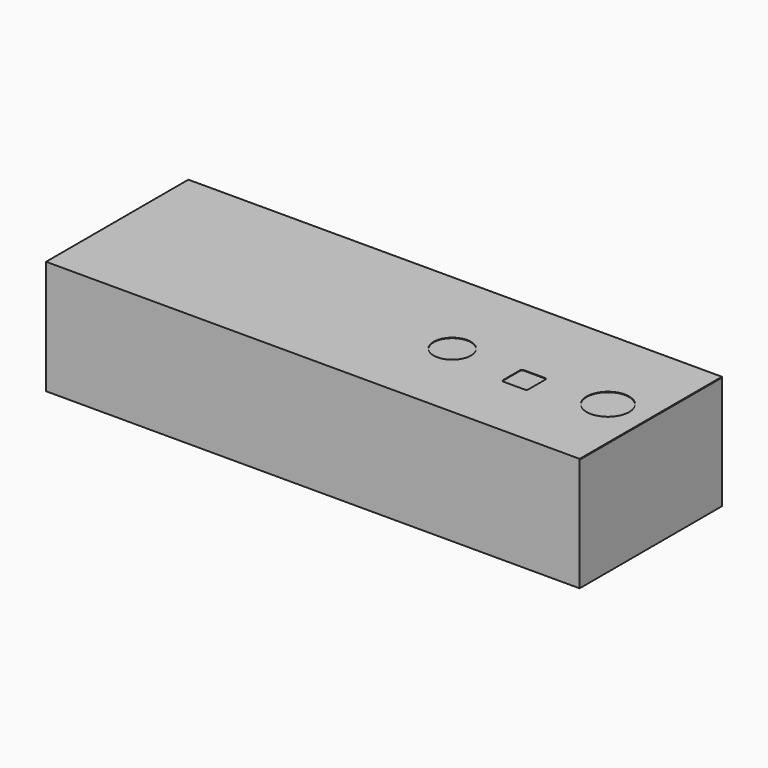
from build123d import *

# Parameters (mm, degrees)
F1_DEPTH = 209.55
F3_DEPTH = 0.4064


# Not quite as in the source:
# - the dataset's text gives a spline's control points without its knots; the knots are read off the source's solid


with BuildPart() as f1:
    # F0 (on Right) → F1 (new body, symmetric)
    with BuildSketch(Plane.YZ):
        Polygon((-139.7, 0), (0, 0), (0, 88.9), (-139.2936, 88.9), (-139.2936, 89.154), (0, 89.154), (0, 89.5604), (-139.7, 89.5604), align=None)
    extrude(amount=F1_DEPTH, both=True)

    # F2 (on face) → F3 (cut, through all)
    with BuildSketch(Plane.XY.offset(89.5604)):
        with BuildLine():
            add(Edge.make_bspline(
                [(107.984345256, -69.4981747566), (107.690467256, -69.7918495566), (107.519068056, -70.2049297566), (107.519068056, -70.6205499566)],
                knots=[1, 1, 1, 1, 2, 2, 2, 2], degree=3))
            Line((107.519068056, -70.6205499566), (107.519068056, -87.2892999566))
            add(Edge.make_bspline(
                [(107.519068056, -87.2892999566), (107.519068056, -87.7047677566), (107.690467256, -88.1178479566), (107.984345256, -88.4117005566)],
                knots=[0, 0, 0, 0, 1, 1, 1, 1], degree=3))
            add(Edge.make_bspline(
                [(107.984345256, -88.4117005566), (108.278197856, -88.7055785566), (108.691278056, -88.8767999566), (109.106568056, -88.8767999566)],
                knots=[1, 1, 1, 1, 2, 2, 2, 2], degree=3))
            Line((109.106568056, -88.8767999566), (125.775318056, -88.8767999566))
            add(Edge.make_bspline(
                [(125.775318056, -88.8767999566), (126.191649456, -88.8767999566), (126.604374056, -88.7055785566), (126.898582256, -88.4117005566)],
                knots=[0, 0, 0, 0, 1, 1, 1, 1], degree=3))
            add(Edge.make_bspline(
                [(126.898582256, -88.4117005566), (127.192130056, -88.1178479566), (127.362818056, -87.7047677566), (127.362818056, -87.2892999566)],
                knots=[1, 1, 1, 1, 2, 2, 2, 2], degree=3))
            Line((127.362818056, -87.2892999566), (127.362818056, -70.6205499566))
            add(Edge.make_bspline(
                [(127.362818056, -70.6205499566), (127.362818056, -70.2049297566), (127.192130056, -69.7918495566), (126.898582256, -69.4981747566)],
                knots=[0, 0, 0, 0, 1, 1, 1, 1], degree=3))
            add(Edge.make_bspline(
                [(126.898582256, -69.4981747566), (126.604374056, -69.2041189566), (126.191649456, -69.0330499566), (125.775318056, -69.0330499566)],
                knots=[1, 1, 1, 1, 2, 2, 2, 2], degree=3))
            Line((125.775318056, -69.0330499566), (109.106568056, -69.0330499566))
            add(Edge.make_bspline(
                [(109.106568056, -69.0330499566), (108.691278056, -69.0330499566), (108.278197856, -69.2041189566), (107.984345256, -69.4981747566)],
                knots=[0, 0, 0, 0, 1, 1, 1, 1], degree=3))
        make_face()
        with BuildLine():
            add(Edge.make_bspline(
                [(67.499971056, -63.8087525566), (64.781434456, -61.0905461566), (60.960512456, -59.5080753566), (57.115943056, -59.5080753566)],
                knots=[7, 7, 7, 7, 8, 8, 8, 8], degree=3))
            add(Edge.make_bspline(
                [(57.115943056, -59.5080753566), (53.272059456, -59.5080753566), (49.451137456, -61.0905461566), (46.732931056, -63.8087525566)],
                knots=[0, 0, 0, 0, 1, 1, 1, 1], degree=3))
            add(Edge.make_bspline(
                [(46.732931056, -63.8087525566), (44.014445256, -66.5272891566), (42.431568056, -70.3477285566), (42.431568056, -74.1924249566), (42.431568056, -78.0366641566), (44.014445256, -81.8574083566), (46.732931056, -84.5756147566)],
                knots=[1, 1, 1, 1, 2, 2, 2, 3, 3, 3, 3], degree=3))
            add(Edge.make_bspline(
                [(46.732931056, -84.5756147566), (49.451137456, -87.2941513566), (53.272059456, -88.8767999566), (57.115943056, -88.8767999566), (60.960512456, -88.8767999566), (64.781434456, -87.2941513566), (67.499971056, -84.5756147566)],
                knots=[3, 3, 3, 3, 4, 4, 4, 5, 5, 5, 5], degree=3))
            add(Edge.make_bspline(
                [(67.499971056, -84.5756147566), (70.218533056, -81.8574083566), (71.800318056, -78.0366641566), (71.800318056, -74.1924249566), (71.800318056, -70.3477285566), (70.218533056, -66.5272891566), (67.499971056, -63.8087525566)],
                knots=[5, 5, 5, 5, 6, 6, 6, 7, 7, 7, 7], degree=3))
        make_face()
        with BuildLine():
            add(Edge.make_bspline(
                [(189.552838456, -60.4213577566), (186.467068656, -57.3355879566), (182.129993256, -55.5393253566), (177.766120856, -55.5393253566)],
                knots=[7, 7, 7, 7, 8, 8, 8, 8], degree=3))
            add(Edge.make_bspline(
                [(177.766120856, -55.5393253566), (173.402223056, -55.5393253566), (169.065198456, -57.3355879566), (165.979758856, -60.4213577566)],
                knots=[0, 0, 0, 0, 1, 1, 1, 1], degree=3))
            add(Edge.make_bspline(
                [(165.979758856, -60.4213577566), (162.894344656, -63.5071275566), (161.097370856, -67.8441775566), (161.097370856, -72.2080499566), (161.097370856, -76.5719477566), (162.894344656, -80.9089977566), (165.979758856, -83.9947675566)],
                knots=[1, 1, 1, 1, 2, 2, 2, 3, 3, 3, 3], degree=3))
            add(Edge.make_bspline(
                [(165.979758856, -83.9947675566), (169.065198456, -87.0801817566), (173.402223056, -88.8767999566), (177.766120856, -88.8767999566), (182.129993256, -88.8767999566), (186.467068656, -87.0801817566), (189.552838456, -83.9947675566)],
                knots=[3, 3, 3, 3, 4, 4, 4, 5, 5, 5, 5], degree=3))
            add(Edge.make_bspline(
                [(189.552838456, -83.9947675566), (192.638582856, -80.9089977566), (194.434870856, -76.5719477566), (194.434870856, -72.2080499566), (194.434870856, -67.8441775566), (192.638582856, -63.5071275566), (189.552838456, -60.4213577566)],
                knots=[5, 5, 5, 5, 6, 6, 6, 7, 7, 7, 7], degree=3))
        make_face()
    extrude(amount=-F3_DEPTH, mode=Mode.SUBTRACT)


solid = f1.part
